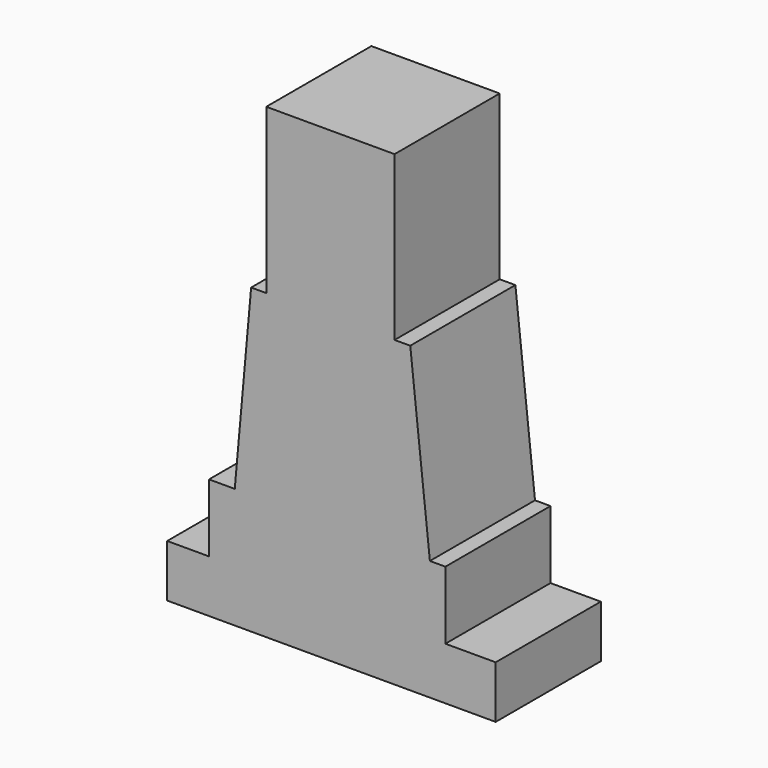
from build123d import *

# Parameters (mm, degrees)
F1_DEPTH = 25.4
F4_DEPTH = 25.4
F5_DEPTH = 25.4


# Not quite as in the source:
# - the program builds the solid bodies; features that only make, move or delete a surface that nothing else refers to are left out


with BuildPart() as f1:
    # F0 (on Front) → F1 (new body)
    with BuildSketch(Plane.XZ):
        Polygon((0, -20.290305838), (0, 0), (-19.4481890649, 0), (-110.8317822218, 0), (-127, 0), (-127, -20.290305838), align=None)
        Polygon((-110.8317822218, 0), (-19.4481890649, 0), (-19.4481890649, 26.2184105814), (-25.4435241222, 26.2184105814), (-100.8837223053, 26.2184105814), (-110.8317822218, 26.2184105814), align=None)
        Polygon((-100.8837223053, 26.2184105814), (-25.4435241222, 26.2184105814), (-33.0289951575, 97.0223118013), (-39.0950739384, 97.0021236187), (-39.0950739384, 96.837057952), (-88.6934632531, 96.837057952), (-94.5519953966, 96.8175604939), align=None)
    extrude(amount=F1_DEPTH)

    # F0 (on Front) → F4 (join)
    with BuildSketch(Plane.XZ):
        Polygon((0, -20.290305838), (0, 0), (-19.4481890649, 0), (-110.8317822218, 0), (-127, 0), (-127, -20.290305838), align=None)
        Polygon((-110.8317822218, 0), (-19.4481890649, 0), (-19.4481890649, 26.2184105814), (-25.4435241222, 26.2184105814), (-100.8837223053, 26.2184105814), (-110.8317822218, 26.2184105814), align=None)
        Polygon((-100.8837223053, 26.2184105814), (-25.4435241222, 26.2184105814), (-33.0289951575, 97.0223118013), (-39.0950739384, 97.0021236187), (-39.0950739384, 96.837057952), (-88.6934632531, 96.837057952), (-94.5519953966, 96.8175604939), align=None)
        Polygon((-39.0950739384, 96.837057952), (-39.0950739384, 97.0021236187), (-88.6934632531, 96.837057952), align=None)
        Polygon((-88.6934632531, 96.837057952), (-39.0950739384, 97.0021236187), (-39.0950739384, 160.250261426), (-88.6934632531, 160.250261426), align=None)
    extrude(amount=F4_DEPTH)

    # F0 (on Front) + F4_face (on face) → F5 (join)
    with BuildSketch(Plane.XZ):
        Polygon((0, -20.290305838), (0, 0), (-19.4481890649, 0), (-110.8317822218, 0), (-127, 0), (-127, -20.290305838), align=None)
        Polygon((-110.8317822218, 0), (-19.4481890649, 0), (-19.4481890649, 26.2184105814), (-25.4435241222, 26.2184105814), (-100.8837223053, 26.2184105814), (-110.8317822218, 26.2184105814), align=None)
        Polygon((-100.8837223053, 26.2184105814), (-25.4435241222, 26.2184105814), (-33.0289951575, 97.0223118013), (-39.0950739384, 97.0021236187), (-39.0950739384, 96.837057952), (-88.6934632531, 96.837057952), (-94.5519953966, 96.8175604939), align=None)
        Polygon((-39.0950739384, 96.837057952), (-39.0950739384, 97.0021236187), (-88.6934632531, 96.837057952), align=None)
        Polygon((-88.6934632531, 96.837057952), (-39.0950739384, 97.0021236187), (-39.0950739384, 160.250261426), (-88.6934632531, 160.250261426), align=None)
    with BuildSketch(Plane(origin=(-63.8821440169, -25.4, 54.1439890392), x_dir=(1, 0, 0), z_dir=(0, -1, 0))):
        Polygon((63.8821440169, -74.4342948772), (63.8821440169, -54.1439890392), (44.433954952, -54.1439890392), (44.433954952, -27.9255784579), (38.4386198947, -27.9255784579), (30.8531488594, 42.8783227621), (24.7870700785, 42.8581345795), (24.7870700785, 106.1062723867), (-24.8113192362, 106.1062723867), (-24.8113192362, 42.6930689128), (-30.6698513797, 42.6735714547), (-37.0015782884, -27.9255784579), (-46.9496382049, -27.9255784579), (-46.9496382049, -54.1439890392), (-63.1178559831, -54.1439890392), (-63.1178559831, -74.4342948772), align=None)
    extrude(amount=F5_DEPTH)


solid = f1.part
